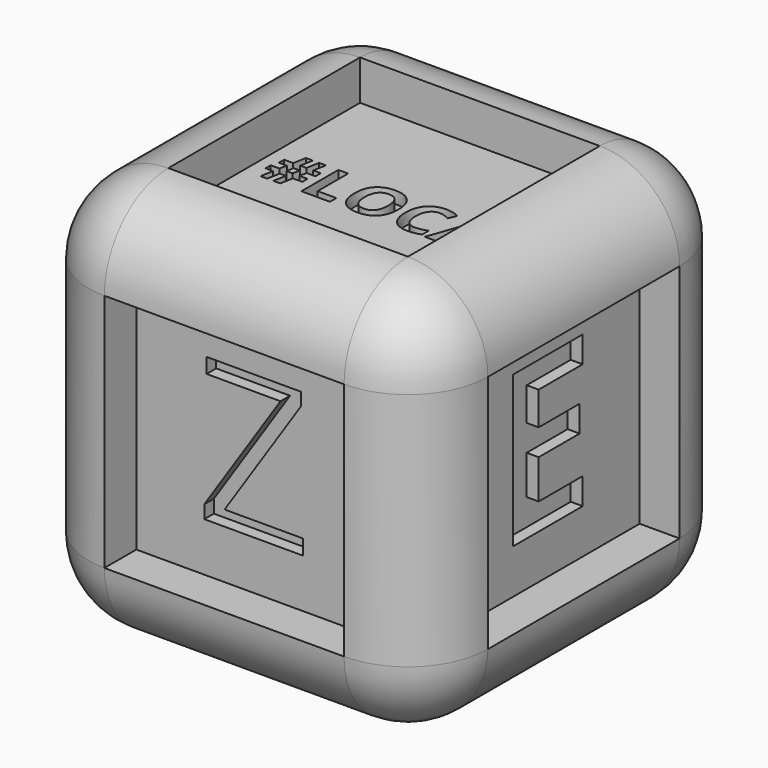
from build123d import *

# Parameters (mm, degrees)
F0_W          = 25.4
F0_H          = 25.4
F1_DEPTH      = 25.4
F2_R          = 5.08
F3_DEPTH      = 2.54
F4_DEPTH      = 2.54
F5_DEPTH      = 2.54
F6_DEPTH      = 5.08
F7_DEPTH      = 2.54
F8_DEPTH      = 2.54
F9_DEPTH      = 5.08
F10_DEPTH     = 2.54
F11_TEXT_SIZE = 12.7932843652
F12_DEPTH     = 0.762
F13_TEXT_SIZE = 13.4681027341
F14_DEPTH     = 0.762
F15_TEXT_SIZE = 13.2270138324
F16_DEPTH     = 0.762
F17_TEXT_SIZE = 12.2133734035
F18_DEPTH     = 0.762
F19_TEXT_SIZE = 4.110145727
F20_DEPTH     = 0.762
F21_TEXT_SIZE = 3.3747782433
F22_DEPTH     = 0.762


# Not quite as in the source:
# - Text() gives the source's letters only with a copy of the font that has no kerning and outlines rounded to 1/6400 em; it was checked with that copy


with BuildPart() as f1:
    # F0 (on Front) → F1 (new body)
    with BuildSketch(Plane.XZ):
        Rectangle(F0_W, F0_H)
    extrude(amount=F1_DEPTH)

    # F2
    f2_edges = [f1.edges().sort_by_distance(p)[0] for p in [
        (-12.7, -25.4, 0),
        (0, -25.4, -12.7),
        (12.7, -25.4, 0),
        (0, -25.4, 12.7),
        (12.7, -12.7, -12.7),
        (12.7, -12.7, 12.7),
        (12.7, 0, 0),
        (-12.7, -12.7, 12.7),
        (0, 0, 12.7),
        (-12.7, 0, 0),
        (0, 0, -12.7),
        (-12.7, -12.7, -12.7),
    ]]
    fillet(f2_edges, radius=F2_R)

    # F3 (cut): a face of the model
    f3_faces = [f1.faces().sort_by_distance(p)[0] for p in [
        (0, -25.4, 0),
    ]]
    extrude(f3_faces, amount=-F3_DEPTH, mode=Mode.SUBTRACT)

    # F4 (cut): a face of the model
    f4_faces = [f1.faces().sort_by_distance(p)[0] for p in [
        (12.7, -12.7, 0),
    ]]
    extrude(f4_faces, amount=-F4_DEPTH, mode=Mode.SUBTRACT)

    # F5 (add): a face of the model
    f5_faces = [f1.faces().sort_by_distance(p)[0] for p in [
        (0, -12.7, 12.7),
    ]]
    extrude(f5_faces, amount=F5_DEPTH)

    # F6 (cut): a face of the model
    f6_faces = [f1.faces().sort_by_distance(p)[0] for p in [
        (0, -12.7, 15.24),
    ]]
    extrude(f6_faces, amount=-F6_DEPTH, mode=Mode.SUBTRACT)

    # F7 (cut): a face of the model
    f7_faces = [f1.faces().sort_by_distance(p)[0] for p in [
        (0, -12.7, -12.7),
    ]]
    extrude(f7_faces, amount=-F7_DEPTH, mode=Mode.SUBTRACT)

    # F8 (add): a face of the model
    f8_faces = [f1.faces().sort_by_distance(p)[0] for p in [
        (0, 0, 0),
    ]]
    extrude(f8_faces, amount=F8_DEPTH)

    # F9 (cut): a face of the model
    f9_faces = [f1.faces().sort_by_distance(p)[0] for p in [
        (0, 2.54, 0),
    ]]
    extrude(f9_faces, amount=-F9_DEPTH, mode=Mode.SUBTRACT)

    # F10 (cut): a face of the model
    f10_faces = [f1.faces().sort_by_distance(p)[0] for p in [
        (-12.7, -12.7, 0),
    ]]
    extrude(f10_faces, amount=-F10_DEPTH, mode=Mode.SUBTRACT)

    # F11 (on face) → F12 (cut)
    with BuildSketch(Plane.XZ.offset(22.86)):
        with Locations((-3.8127286353, -4.5142196139)):
            Text('Z', F11_TEXT_SIZE, font='Open Sans', text_align=(TextAlign.LEFT, TextAlign.BOTTOM))
    extrude(amount=-F12_DEPTH, mode=Mode.SUBTRACT)

    # F13 (on face) → F14 (cut)
    with BuildSketch(Plane.YZ.offset(10.16)):
        with Locations((-16.3566274694, -4.7961947009)):
            Text('E', F13_TEXT_SIZE, font='Open Sans', font_style=FontStyle.BOLD, text_align=(TextAlign.LEFT, TextAlign.BOTTOM))
    extrude(amount=-F14_DEPTH, mode=Mode.SUBTRACT)

    # F15 (on face) → F16 (cut)
    with BuildSketch(Plane(origin=(0, -2.54, 0), x_dir=(-1, 0, 0), z_dir=(0, 1, 0))):
        with Locations((-3.8633323579, -4.5891155475)):
            Text('S', F15_TEXT_SIZE, font='Open Sans', font_style=FontStyle.BOLD, text_align=(TextAlign.LEFT, TextAlign.BOTTOM))
    extrude(amount=-F16_DEPTH, mode=Mode.SUBTRACT)

    # F17 (on face) → F18 (cut)
    with BuildSketch(Plane(origin=(-10.16, 0, 0), x_dir=(0, -1, 0), z_dir=(-1, 0, 0))):
        with Locations((9.0334945054, -4.1014490234)):
            Text('T', F17_TEXT_SIZE, font='Open Sans', font_style=FontStyle.BOLD, text_align=(TextAlign.LEFT, TextAlign.BOTTOM))
    extrude(amount=-F18_DEPTH, mode=Mode.SUBTRACT)

    # F19 (on face) → F20 (cut)
    with BuildSketch(Plane.XY.offset(10.16)):
        with Locations((-6.9772160175, -14.3240965965)):
            Text('#LOCA', F19_TEXT_SIZE, font='Open Sans', font_style=FontStyle.BOLD, text_align=(TextAlign.LEFT, TextAlign.BOTTOM))
    extrude(amount=-F20_DEPTH, mode=Mode.SUBTRACT)

    # F21 (on face) → F22 (cut)
    with BuildSketch(Plane(origin=(0, 0, -10.16), x_dir=(1, 0, 0), z_dir=(0, 0, -1))):
        with Locations((-6.9753618121, 11.803623791)):
            Text('Just Live.', F21_TEXT_SIZE, font='Open Sans', text_align=(TextAlign.LEFT, TextAlign.BOTTOM))
    extrude(amount=-F22_DEPTH, mode=Mode.SUBTRACT)


solid = f1.part
